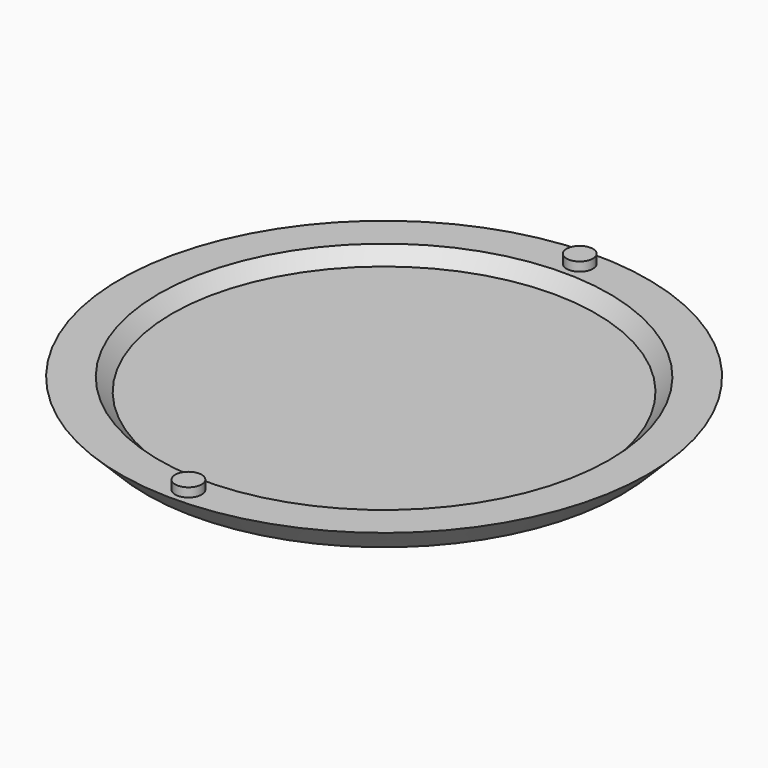
from build123d import *

# Parameters (mm, degrees)
F0_R      = 50.8
F1_DEPTH  = 38.1
F1_TAPER  = 35
F2_R      = 44.45
F3_DEPTH  = 31.75
F3_TAPER  = 35
F6_R      = 6.35
F13_W     = 40.0871150196
F13_H     = 221.6413393617
F14_DEPTH = 38.1
F16_R     = 63.4410735664
F17_DEPTH = 6.35
F17_TAPER = 45
F18_R     = 54.1198096159
F19_DEPTH = 3.175
F19_TAPER = 45
F20_R     = 2.38125
F21_DEPTH = 6.35
F23_W     = 544.7718501091
F23_H     = 283.927500248
F24_DEPTH = 65.204810909
F25_R     = 3.175
F26_DEPTH = 2.159


# Not quite as in the source:
# - a feature of the source that left no trace in its solid (it failed there, or was rolled back) is left out
# - a feature names something its author has since deleted; it is built from what else it names


with BuildPart() as f1:
    # F0 (on Top) → F1 (new body)
    with BuildSketch(Plane.XY):
        Circle(F0_R)
    extrude(amount=-F1_DEPTH, taper=F1_TAPER)

    # F2 (on face) → F3 (cut)
    with BuildSketch(Plane.XY):
        Circle(F2_R)
    extrude(amount=-F3_DEPTH, taper=F3_TAPER, mode=Mode.SUBTRACT)

    # F9: F7 across plane


with BuildPart() as f7:
    # F7: sweep along a path in F4
    with BuildLine(Plane.YZ) as f7_path:
        add(Plane.YZ * Edge.make_bspline(
            [(-50.8, 0), (-59.5457513783, -8.9993874064), (-82.8005315743, -30.8254243712), (-59.2938947205, -72.9983075974), (-50.8, -97.5854156721)],
            knots=[0, 0, 0, 0, 0.421582605, 1, 1, 1, 1], degree=3))
    # F6 (on plane+point) → F7 (sweep)
    with BuildSketch(Plane.XZ.offset(50.8)):
        with Locations((0, -6.35)):
            Circle(F6_R)
    sweep(path=f7_path.line)


with BuildPart() as f1_1:
    add(f1.part)
    add(f7.part.mirror(Plane.XZ))


with BuildPart() as f14_tool:
    # F13 (on plane+point) → F14 (new body)
    with BuildSketch(Plane.XY.offset(-103.303810809)):
        with Locations((2.3701563478, 10.5300284922)):
            Rectangle(F13_W, F13_H)
    extrude(amount=F14_DEPTH)


with BuildPart() as f1_2:
    add(f1_1.part)

    # F14: cut by f14_tool
    add(f14_tool.part, mode=Mode.SUBTRACT)



with BuildPart() as f7_1:
    add(f7.part)

    # F14: cut by f14_tool
    add(f14_tool.part, mode=Mode.SUBTRACT)


with BuildPart() as f1_3:
    add(f1_2.part)

    add(f7_1.part)  # F17 merges F7
    # F16 (on face) → F17 (join)
    with BuildSketch(Plane(origin=(0, 0, -65.203810809), x_dir=(1, 0, 0), z_dir=(0, 0, -1))):
        Circle(F16_R)
    extrude(amount=F17_DEPTH, taper=F17_TAPER)

    # F18 (on face) → F19 (cut)
    with BuildSketch(Plane.XY.offset(-65.203810809)):
        Circle(F18_R)
    extrude(amount=-F19_DEPTH, taper=F19_TAPER, mode=Mode.SUBTRACT)

    # F20 (on face) → F21 (cut, through all)
    with BuildSketch(Plane.XY.offset(-31.75)):
        Circle(F20_R)
    extrude(amount=-F21_DEPTH, mode=Mode.SUBTRACT)

    # F23 (on offset) → F24 (cut, through all)
    with BuildSketch(Plane.XY.offset(-65.203810809)):
        Rectangle(F23_W, F23_H)
    extrude(amount=F24_DEPTH, mode=Mode.SUBTRACT)

    # F25 (on face) → F26 (join)
    with BuildSketch(Plane.XY.offset(-65.203810809)):
        with Locations((0, 58.78068)):
            Circle(F25_R)
    f26 = extrude(amount=F26_DEPTH)

    # F27: F26 across plane
    add(f26.mirror(Plane.XZ))


solid = f1_3.part
